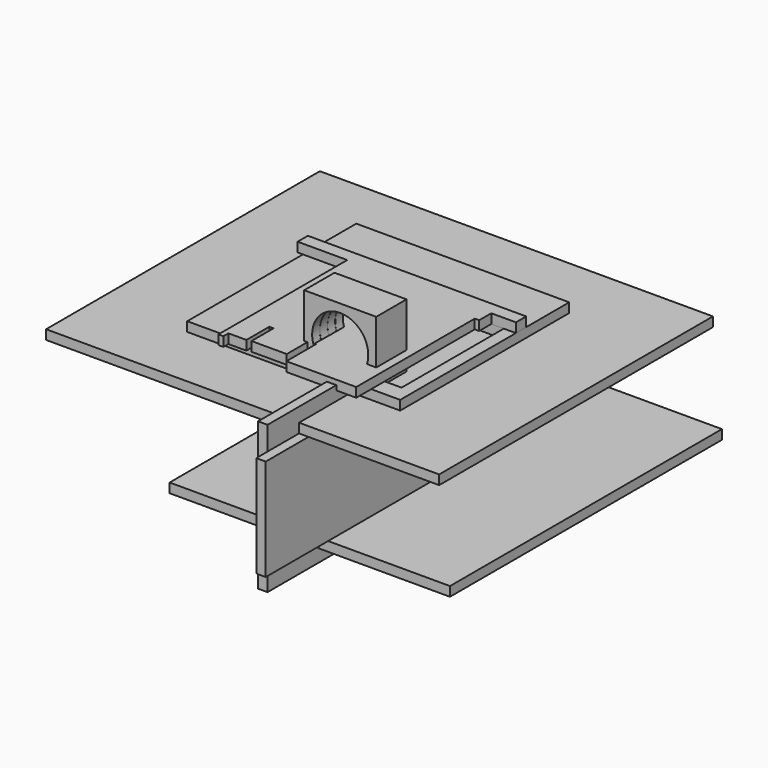
from build123d import *

# Parameters (mm, degrees)
F0_W      = 193.3809220791
F0_H      = 196.0519328713
F0_R      = 74.8892897361
F1_DEPTH  = 25.4
F2_W      = 193.3809220791
F2_H      = 196.0519328713
F2_R      = 74.655991807
F3_DEPTH  = 25.4
F4_W      = 176.1402115226
F4_H      = 196.0519328713
F4_R      = 74.3860816692
F4_W_2    = 17.2407105565
F5_DEPTH  = 25.4
F6_W      = 193.3809220791
F6_H      = 196.0519328713
F6_R      = 75.3545401658
F7_DEPTH  = 25.4
F8_W      = 193.4532523155
F8_H      = 35.7192189813
F9_DEPTH  = 25.4
F11_DEPTH = 404.6249985695
F12_W     = 1055.474460125
F12_H     = 918.9680218697
F13_DEPTH = 25.4
F14_W     = 752.8154850006
F14_H     = 912.7593636513
F15_DEPTH = 25.4
F16_W     = 870.2914460182
F16_H     = 272.9075178504
F17_DEPTH = 25.4
F18_W     = 400.6907343864
F18_H     = 395.6300988793
F19_DEPTH = 25.4
F20_W     = 571.7930793762
F20_H     = 567.36561656
F21_DEPTH = 25.4
F23_W     = 78.0102312565
F23_H     = 34.4761013985
F23_W_2   = 13.3122801781
F23_H_2   = 332.7346146107
F23_W_3   = 187.4931752682
F23_H_3   = 105.7706475258
F23_H_4   = 99.6497869492
F24_DEPTH = 25.4
F25_W     = 101.5389561653
F25_H     = 251.5766620636
F25_H_2   = 50.2630472183
F25_W_2   = 29.5691788197
F25_W_3   = 54.5960366726
F25_H_3   = 76.733738184
F26_DEPTH = 25.4


with BuildPart() as f1:
    # F0 (on Front) → F1 (new body)
    with BuildSketch(Plane.XZ):
        with Locations((-0.0024288893, -0.3737099469)):
            Rectangle(F0_W, F0_H)
        Circle(F0_R, mode=Mode.SUBTRACT)
    extrude(amount=F1_DEPTH)

    # F2 (on face) → F3 (join)
    with BuildSketch(Plane(origin=(0, 0, 0), x_dir=(-1, 0, 0), z_dir=(0, 1, 0))):
        with Locations((0.0024288893, -0.3737099469)):
            Rectangle(F2_W, F2_H)
        Circle(F2_R, mode=Mode.SUBTRACT)
    extrude(amount=F3_DEPTH)

    # F4 (on face) → F5 (join)
    with BuildSketch(Plane(origin=(0, 25.4, 0), x_dir=(-1, 0, 0), z_dir=(0, 1, 0))):
        with Locations((-8.617926389, -0.3737099469)):
            Rectangle(F4_W, F4_H)
        Circle(F4_R, mode=Mode.SUBTRACT)
        with Locations((88.0725346506, -0.3737099469)):
            Rectangle(F4_W_2, F4_H)
    extrude(amount=F5_DEPTH)

    # F6 (on face) → F7 (join)
    with BuildSketch(Plane.XZ.offset(25.4)):
        with Locations((-0.0024288893, -0.3737099469)):
            Rectangle(F6_W, F6_H)
        Circle(F6_R, mode=Mode.SUBTRACT)
    extrude(amount=F7_DEPTH)

    # F8 (on face) → F9 (join)
    with BuildSketch(Plane(origin=(0, 0, -98.3996763825), x_dir=(1, 0, 0), z_dir=(0, 0, -1))):
        with Locations((0.0337362289, 68.6596094906)):
            Rectangle(F8_W, F8_H)
        Polygon((96.7603623867, 50.8), (-96.6928899288, 50.8), (-97.9034900665, 50.8), (-97.9034900665, -97.2673520446), (96.7603623867, -97.2673520446), align=None)
    extrude(amount=F9_DEPTH)

    # F10 (on face) → F11 (join)
    with BuildSketch(Plane(origin=(0, 50.8, 0), x_dir=(-1, 0, 0), z_dir=(0, 1, 0))):
        Polygon((-65.7769590616, -350.3327965736), (-65.7769590616, -371.3071942329), (119.0916895866, -371.3071942329), (119.0916895866, -98.3996763825), (-65.7769590616, -98.3996763825), align=None)
    extrude(amount=F11_DEPTH)

    # F12 (on face) → F13 (join)
    with BuildSketch(Plane.XY.offset(-98.3996763825)):
        with Locations((-85.7326686382, 188.2182061672)):
            Rectangle(F12_W, F12_H)
    extrude(amount=F13_DEPTH)

    # F14 (on face) → F15 (join)
    with BuildSketch(Plane(origin=(0, 0, -371.3071942329), x_dir=(1, 0, 0), z_dir=(0, 0, -1))):
        with Locations((42.0474410057, -250.8960068226)):
            Rectangle(F14_W, F14_H)
    extrude(amount=F15_DEPTH)

    # F16 (on face) → F17 (join)
    with BuildSketch(Plane.YZ.offset(65.7769590616)):
        with Locations((20.2792755604, -234.8534353077)):
            Rectangle(F16_W, F16_H)
    extrude(amount=F17_DEPTH)

    # F18 (on face) → F19 (join)
    with BuildSketch(Plane(origin=(65.7769590616, 0, 0), x_dir=(0, -1, 0), z_dir=(-1, 0, 0))):
        with Locations((176.6569912434, -232.9259328544)):
            Rectangle(F18_W, F18_H)
    extrude(amount=F19_DEPTH)

    # F20 (on face) → F21 (join)
    with BuildSketch(Plane.XY.offset(-72.9996763825)):
        with Locations((-88.7070894241, 187.6235455275)):
            Rectangle(F20_W, F20_H)
        Polygon((40.3769590616, -50.8), (-18.691013125, -50.8), (-18.691013125, 275.1325964928), (-18.691013125, 292.6656007767), (40.3769590616, 292.6656007767), (164.7324860096, 292.6656007767), (164.7324860096, -50.8), (129.8503279686, -50.8), align=None, mode=Mode.SUBTRACT)
    extrude(amount=F21_DEPTH)

    # F23 (on face) → F24 (join)
    with BuildSketch(Plane.XY.offset(-47.5996763825)):
        Polygon((119.2969679832, -40.3836667538), (119.2969679832, 292.3509478569), (-242.377102375, 292.3509478569), (-242.377102375, -40.3836667538), (-68.1962072849, -40.3836667538), align=None)
        with Locations((158.3020836115, 309.5889985561)):
            Rectangle(F23_W, F23_H)
        Polygon((-242.377102375, 292.3509478569), (119.2969679832, 292.3509478569), (119.2969679832, 326.8270492554), (-389.0109658241, 326.8270492554), (-389.0109658241, 292.3509478569), (-255.6893825531, 292.3509478569), align=None)
        with Locations((-249.0332424641, 125.9836405516)):
            Rectangle(F23_W_2, F23_H_2)
        with Locations((25.5503803492, -93.2689905167)):
            Rectangle(F23_W_3, F23_H_3)
        with Locations((-249.0332424641, -90.2085602283)):
            Rectangle(F23_W_2, F23_H_4)
    extrude(amount=F24_DEPTH)

    # F25 (on face) → F26 (join)
    with BuildSketch(Plane.XY.offset(-47.5996763825)):
        Polygon((101.5389561653, 0), (0, 0), (-69.8948949575, 0), (-69.8948949575, -46.3175177574), (101.5389561653, -46.3175177574), align=None)
        Polygon((-69.8948949575, 0), (0, 0), (0, 251.5766620636), (0, 301.8397092819), (-69.8948949575, 301.8397092819), (-69.8948949575, 239.4688427448), align=None)
        with Locations((50.7694780827, 125.7883310318)):
            Rectangle(F25_W, F25_H)
        Polygon((-69.8948949575, -46.3175177574), (-69.8948949575, 0), (-69.8948949575, 239.4688427448), (-116.5921464562, 239.4688427448), (-116.5921464562, -46.3175177574), (-88.026702404, -46.3175177574), align=None)
        with Locations((50.7694780827, 276.7081856728)):
            Rectangle(F25_W, F25_H_2)
        Polygon((-116.5921464562, 239.4688427448), (-69.8948949575, 239.4688427448), (-69.8948949575, 301.8397092819), (-248.7161755562, 301.8397092819), (-248.7161755562, 239.4688427448), align=None)
        with Locations((116.3235455751, 276.7081856728)):
            Rectangle(F25_W_2, F25_H_2)
        Polygon((-116.5921464562, -46.3175177574), (-116.5921464562, 239.4688427448), (-248.7161755562, 239.4688427448), (-248.7161755562, -46.3175177574), (-194.1201388836, -46.3175177574), (-182.6541610062, -46.3175177574), align=None)
        Polygon((-88.026702404, -120.3344464302), (-88.026702404, -46.3175177574), (-116.5921464562, -46.3175177574), (-182.6541610062, -46.3175177574), (-182.6541610062, -120.3344464302), align=None)
        with Locations((-221.4181572199, -84.6843868494)):
            Rectangle(F25_W_3, F25_H_3)
    extrude(amount=F26_DEPTH)


solid = f1.part
